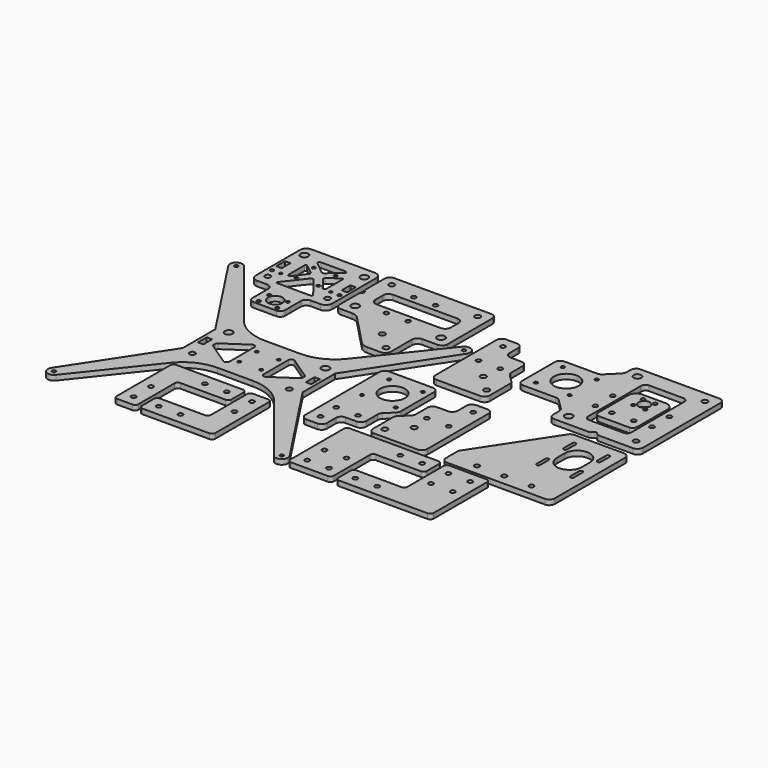
from build123d import *

# Parameters (mm, degrees)
F0_R     = 1.55
F0_R_2   = 6.75
F0_R_3   = 2.55
F0_R_4   = 1.6
F0_R_5   = 1.25
F0_R_6   = 1.5
F0_W     = 5
F0_H     = 10
F0_R_7   = 3.556
F1_DEPTH = 2.325
F0_R_8   = 2.15
F0_R_9   = 2.1
F0_R_10  = 11.5
F0_R_11  = 2.6
F0_R_12  = 1.65
F0_R_13  = 3.555
F0_R_14  = 2.125
F0_R_15  = 1.7531
F0_R_16  = 5.2592
F0_R_17  = 2.25


# Not quite as in the source:
# - ends of sketch curves that miss each other by under 0.0002 mm in the source are joined


with BuildPart() as f1:
    # F0 (on Top) → F1 (new body, symmetric)
    with BuildSketch(Plane.XY):
        with BuildLine():
            ThreePointArc((-173.037736, 133.310467), (-177.2803766871, 131.5531076871), (-179.037736, 127.310467))
            Line((-179.037736, 127.310467), (-179.037736, 76.929897))
            ThreePointArc((-179.037736, 76.929897), (-177.2803766871, 72.6872563129), (-173.037736, 70.929897))
            Line((-173.037736, 70.929897), (-164.037736, 70.929897))
            ThreePointArc((-164.037736, 70.929897), (-160.5022020941, 69.4654309059), (-159.037736, 65.929897))
            Line((-159.037736, 65.929897), (-159.037736, 47.929897))
            ThreePointArc((-159.037736, 47.929897), (-157.7197165153, 44.7479164847), (-154.537736, 43.429897))
            Line((-154.537736, 43.429897), (-133.537736, 43.429897))
            ThreePointArc((-133.537736, 43.429897), (-130.3557554847, 44.7479164847), (-129.037736, 47.929897))
            Line((-129.037736, 47.929897), (-129.037736, 65.929897))
            ThreePointArc((-129.037736, 65.929897), (-127.5732699059, 69.4654309059), (-124.037736, 70.929897))
            Line((-124.037736, 70.929897), (-115.037736, 70.929897))
            ThreePointArc((-115.037736, 70.929897), (-110.7950953129, 72.6872563129), (-109.037736, 76.929897))
            Line((-109.037736, 76.929897), (-109.037736, 127.310467))
            ThreePointArc((-109.037736, 127.310467), (-110.7950953129, 131.5531076871), (-115.037736, 133.310467))
            Line((-115.037736, 133.310467), (-173.037736, 133.310467))
        make_face()
        with Locations((-152.537736, 47.029897)):
            Circle(F0_R, mode=Mode.SUBTRACT)
        with Locations((-135.537736, 47.029897)):
            Circle(F0_R, mode=Mode.SUBTRACT)
        with Locations((-152.537736, 59.029897)):
            Circle(F0_R, mode=Mode.SUBTRACT)
        with Locations((-144.037736, 55.429897)):
            Circle(F0_R_2, mode=Mode.SUBTRACT)
        with Locations((-135.537736, 59.029897)):
            Circle(F0_R, mode=Mode.SUBTRACT)
        with Locations((-171.537736, 81.114382)):
            Circle(F0_R_3, mode=Mode.SUBTRACT)
        with Locations((-174.992762, 90.275039)):
            Circle(F0_R_4, mode=Mode.SUBTRACT)
        with Locations((-166.992762, 90.275039)):
            Circle(F0_R_5, mode=Mode.SUBTRACT)
        with Locations((-154.037736, 92.120182)):
            Circle(F0_R_6, mode=Mode.SUBTRACT)
        with BuildLine():
            Line((-161.537736, 92.349506), (-161.537736, 110.969423))
            ThreePointArc((-161.537736, 110.969423), (-160.9765059421, 111.8680224313), (-159.9227741241, 111.7579798408))
            Line((-159.9227741241, 111.7579798408), (-150.887467, 104.711742))
            ThreePointArc((-150.887467, 104.711742), (-150.3212527314, 103.7130323531), (-150.6270730647, 102.6064640505))
            Line((-150.6270730647, 102.6064640505), (-151.006303, 102.120182))
            Line((-151.006303, 102.120182), (-158.828462, 91.462006))
            ThreePointArc((-158.828462, 91.462006), (-160.5046883222, 90.9240392242), (-161.537736, 92.349506))
        make_face(mode=Mode.SUBTRACT)
        with Locations((-116.537736, 81.114382)):
            Circle(F0_R_3, mode=Mode.SUBTRACT)
        with BuildLine():
            Line((-128.58573, 76.929897), (-159.489741, 76.929897))
            ThreePointArc((-159.489741, 76.929897), (-160.3883402583, 77.4911267036), (-160.2782983258, 78.544858254))
            Line((-160.2782983258, 78.544858254), (-145.61485, 97.347622))
            ThreePointArc((-145.61485, 97.347622), (-144.0377356925, 98.1177), (-142.4606209703, 97.3476220232))
            Line((-142.4606209703, 97.3476220232), (-127.797173, 78.544858))
            ThreePointArc((-127.797173, 78.544858), (-127.6871307417, 77.4911267036), (-128.58573, 76.929897))
        make_face(mode=Mode.SUBTRACT)
        with Locations((-134.037736, 92.120182)):
            Circle(F0_R_6, mode=Mode.SUBTRACT)
        with BuildLine():
            Line((-129.220572, 91.210621), (-137.85836, 102.286753))
            ThreePointArc((-137.85836, 102.286753), (-138.1641792309, 103.3933216583), (-137.5979649495, 104.3920309353))
            Line((-137.5979649495, 104.3920309353), (-128.152697, 111.75798))
            ThreePointArc((-128.152697, 111.75798), (-127.0989657036, 111.8680222583), (-126.537736, 110.969423))
            Line((-126.537736, 110.969423), (-126.537736, 92.133063))
            ThreePointArc((-126.537736, 92.133063), (-127.5500136932, 90.7145683925), (-129.220572, 91.210621))
        make_face(mode=Mode.SUBTRACT)
        with Locations((-120.992762, 90.275039)):
            Circle(F0_R_5, mode=Mode.SUBTRACT)
        with Locations((-112.992762, 90.275039)):
            Circle(F0_R_4, mode=Mode.SUBTRACT)
        with Locations((-174.037736, 102.120182)):
            Rectangle(F0_W, F0_H, mode=Mode.SUBTRACT)
        with Locations((-154.037736, 112.120182)):
            Circle(F0_R_6, mode=Mode.SUBTRACT)
        with Locations((-171.537736, 123.125982)):
            Circle(F0_R_7, mode=Mode.SUBTRACT)
        with BuildLine():
            Line((-155.334091, 121.809978), (-132.741381, 121.809978))
            ThreePointArc((-132.741381, 121.809978), (-131.3304796262, 120.8192493553), (-131.7833387935, 119.1557877512))
            Line((-131.7833387935, 119.1557877512), (-142.760347, 110.044269))
            ThreePointArc((-142.760347, 110.044269), (-144.0377356153, 109.58319), (-145.3151243278, 110.044268605))
            Line((-145.3151243278, 110.044268605), (-156.292132, 119.155788))
            ThreePointArc((-156.292132, 119.155788), (-156.7449925044, 120.8192489935), (-155.334091, 121.809978))
        make_face(mode=Mode.SUBTRACT)
        with Locations((-134.037736, 112.120182)):
            Circle(F0_R_6, mode=Mode.SUBTRACT)
        with Locations((-114.037736, 102.120182)):
            Rectangle(F0_W, F0_H, mode=Mode.SUBTRACT)
        with Locations((-116.537736, 123.125982)):
            Circle(F0_R_7, mode=Mode.SUBTRACT)
    extrude(amount=F1_DEPTH, both=True)


with BuildPart() as f1b:
    # F0 (on Top) → F1, piece 2 (new body, symmetric)
    with BuildSketch(Plane.XY):
        with BuildLine():
            Line((-116.875232, -87.385385), (-75.37523, -87.385385))
            ThreePointArc((-75.37523, -87.385385), (-73.2539096564, -86.5067053436), (-72.37523, -84.385385))
            Line((-72.37523, -84.385385), (-72.37523, -70.385385))
            ThreePointArc((-72.37523, -70.385385), (-73.2539096564, -68.2640646564), (-75.37523, -67.385385))
            Line((-75.37523, -67.385385), (-136.87523, -67.385385))
            ThreePointArc((-136.87523, -67.385385), (-138.9965503436, -68.2640646564), (-139.87523, -70.385385))
            Line((-139.87523, -70.385385), (-139.87523, -131.885385))
            ThreePointArc((-139.87523, -131.885385), (-138.9965503436, -134.0067053436), (-136.87523, -134.885385))
            Line((-136.87523, -134.885385), (-122.875232, -134.885385))
            ThreePointArc((-122.875232, -134.885385), (-120.7539116564, -134.0067053436), (-119.875232, -131.885385))
            Line((-119.875232, -131.885385), (-119.875232, -90.385385))
            ThreePointArc((-119.875232, -90.385385), (-118.9965523436, -88.2640646564), (-116.875232, -87.385385))
        make_face()
        with Locations((-129.875231, -124.885385)):
            Circle(F0_R_8, mode=Mode.SUBTRACT)
        with Locations((-129.875231, -104.885385)):
            Circle(F0_R_8, mode=Mode.SUBTRACT)
        with Locations((-102.37523, -77.385385)):
            Circle(F0_R_8, mode=Mode.SUBTRACT)
        with Locations((-82.37523, -77.385385)):
            Circle(F0_R_8, mode=Mode.SUBTRACT)
    extrude(amount=F1_DEPTH, both=True)


with BuildPart() as f1c:
    # F0 (on Top) → F1, piece 3 (new body, symmetric)
    with BuildSketch(Plane.XY):
        with BuildLine():
            ThreePointArc((-51.875233, -135.385385), (-49.7539126564, -134.5067053436), (-48.875233, -132.385385))
            Line((-48.875233, -132.385385), (-48.875233, -70.885386))
            ThreePointArc((-48.875233, -70.885386), (-49.7539126564, -68.7640656564), (-51.875233, -67.885386))
            Line((-51.875233, -67.885386), (-65.875232, -67.885386))
            ThreePointArc((-65.875232, -67.885386), (-67.9965523436, -68.7640656564), (-68.875232, -70.885386))
            Line((-68.875232, -70.885386), (-68.875232, -112.385385))
            ThreePointArc((-68.875232, -112.385385), (-69.7539116564, -114.5067053436), (-71.875232, -115.385385))
            Line((-71.875232, -115.385385), (-113.375233, -115.385385))
            ThreePointArc((-113.375233, -115.385385), (-115.4965533436, -116.2640646564), (-116.375233, -118.385385))
            Line((-116.375233, -118.385385), (-116.375233, -132.385385))
            ThreePointArc((-116.375233, -132.385385), (-115.4965533436, -134.5067053436), (-113.375233, -135.385385))
            Line((-113.375233, -135.385385), (-51.875233, -135.385385))
        make_face()
        with Locations((-106.375233, -125.385385)):
            Circle(F0_R_8, mode=Mode.SUBTRACT)
        with Locations((-86.375233, -125.385385)):
            Circle(F0_R_8, mode=Mode.SUBTRACT)
        with Locations((-58.875232, -97.885386)):
            Circle(F0_R_8, mode=Mode.SUBTRACT)
        with Locations((-58.875232, -77.885386)):
            Circle(F0_R_8, mode=Mode.SUBTRACT)
    extrude(amount=F1_DEPTH, both=True)


with BuildPart() as f1d:
    # F0 (on Top) → F1, piece 4 (new body, symmetric)
    with BuildSketch(Plane.XY):
        with BuildLine():
            Line((33.884182, -23.014414), (33.884182, 14.914518))
            ThreePointArc((33.884182, 14.914518), (32.4197159059, 18.4500519059), (28.884182, 19.914518))
            Line((28.884182, 19.914518), (-11.115818, 19.914518))
            ThreePointArc((-11.115818, 19.914518), (-14.6513519059, 18.4500519059), (-16.115818, 14.914518))
            Line((-16.115818, 14.914518), (-16.115818, -70.085482))
            ThreePointArc((-16.115818, -70.085482), (-14.6513519059, -73.6210159059), (-11.115818, -75.085482))
            Line((-11.115818, -75.085482), (-1.115818, -75.085482))
            ThreePointArc((-1.115818, -75.085482), (2.4197159059, -73.6210159059), (3.884182, -70.085482))
            Line((3.884182, -70.085482), (3.884182, -60.085482))
            ThreePointArc((3.884182, -60.085482), (5.3486480941, -56.5499480941), (8.884182, -55.085482))
            Line((8.884182, -55.085482), (18.884182, -55.085482))
            ThreePointArc((18.884182, -55.085482), (22.4197159059, -53.6210159059), (23.884182, -50.085482))
            Line((23.884182, -50.085482), (23.884182, -37.15655))
            ThreePointArc((23.884182, -37.15655), (24.2647843374, -35.2431328382), (25.3486480941, -33.6210160941))
            Line((25.3486480941, -33.6210160941), (32.419716, -26.549948))
            ThreePointArc((32.419716, -26.549948), (33.5035796626, -24.9278311618), (33.884182, -23.014414))
        make_face()
        with Locations((-6.115818, -65.085482)):
            Circle(F0_R_9, mode=Mode.SUBTRACT)
        with Locations((-6.115818, -47.085482)):
            Circle(F0_R_9, mode=Mode.SUBTRACT)
        with Locations((-3.615818, -20.585482)):
            Circle(F0_R_4, mode=Mode.SUBTRACT)
        with Locations((13.884182, -47.085482)):
            Circle(F0_R_9, mode=Mode.SUBTRACT)
        with Locations((27.384182, -20.585482)):
            Circle(F0_R_4, mode=Mode.SUBTRACT)
        with Locations((11.884182, -5.085482)):
            Circle(F0_R_10, mode=Mode.SUBTRACT)
        with Locations((-3.615818, 10.414518)):
            Circle(F0_R_4, mode=Mode.SUBTRACT)
        with Locations((27.384182, 10.414518)):
            Circle(F0_R_4, mode=Mode.SUBTRACT)
    extrude(amount=F1_DEPTH, both=True)


with BuildPart() as f1e:
    # F0 (on Top) → F1, piece 5 (new body, symmetric)
    with BuildSketch(Plane.XY):
        with BuildLine():
            Line((45.248714, -6.784818), (45.248714, -19.713751))
            ThreePointArc((45.248714, -19.713751), (44.8681117979, -21.6271678352), (43.7842484059, -23.2492844059))
            Line((43.7842484059, -23.2492844059), (36.71318, -30.320352))
            ThreePointArc((36.71318, -30.320352), (35.6293163374, -31.9424688382), (35.248714, -33.855886))
            Line((35.248714, -33.855886), (35.248714, -56.784818))
            ThreePointArc((35.248714, -56.784818), (36.7131800941, -60.3203519059), (40.248714, -61.784818))
            Line((40.248714, -61.784818), (80.248714, -61.784818))
            ThreePointArc((80.248714, -61.784818), (83.7842479059, -60.3203519059), (85.248714, -56.784818))
            Line((85.248714, -56.784818), (85.248714, 13.215182))
            ThreePointArc((85.248714, 13.215182), (83.7842479059, 16.7507159059), (80.248714, 18.215182))
            Line((80.248714, 18.215182), (70.248714, 18.215182))
            ThreePointArc((70.248714, 18.215182), (66.7131800941, 16.7507159059), (65.248714, 13.215182))
            Line((65.248714, 13.215182), (65.248714, 3.215182))
            ThreePointArc((65.248714, 3.215182), (63.7842479059, -0.3203519059), (60.248714, -1.784818))
            Line((60.248714, -1.784818), (50.248714, -1.784818))
            ThreePointArc((50.248714, -1.784818), (46.7131800941, -3.2492840941), (45.248714, -6.784818))
        make_face()
        with Locations((42.248714, -51.784818)):
            Circle(F0_R_11, mode=Mode.SUBTRACT)
        with Locations((57.248714, -36.784818)):
            Circle(F0_R_11, mode=Mode.SUBTRACT)
        with Locations((55.248714, -19.784818)):
            Circle(F0_R_9, mode=Mode.SUBTRACT)
        with Locations((75.248714, -19.784818)):
            Circle(F0_R_9, mode=Mode.SUBTRACT)
        with Locations((75.248714, 8.215182)):
            Circle(F0_R_9, mode=Mode.SUBTRACT)
    extrude(amount=F1_DEPTH, both=True)


with BuildPart() as f1f:
    # F0 (on Top) → F1, piece 6 (new body, symmetric)
    with BuildSketch(Plane.XY):
        with BuildLine():
            Line((68.248714, 36.215182), (68.248714, 59.144114))
            ThreePointArc((68.248714, 59.144114), (67.8681116626, 61.0575311618), (66.7842479059, 62.6796479059))
            Line((66.7842479059, 62.6796479059), (59.71318, 69.750716))
            ThreePointArc((59.71318, 69.750716), (58.6293162021, 71.3728321648), (58.248714, 73.286249))
            Line((58.248714, 73.286249), (58.248714, 86.215182))
            ThreePointArc((58.248714, 86.215182), (56.7842479059, 89.7507159059), (53.248714, 91.215182))
            Line((53.248714, 91.215182), (43.248714, 91.215182))
            ThreePointArc((43.248714, 91.215182), (39.7131800941, 92.6796480941), (38.248714, 96.215182))
            Line((38.248714, 96.215182), (38.248714, 106.215182))
            ThreePointArc((38.248714, 106.215182), (36.7842479059, 109.7507159059), (33.248714, 111.215182))
            Line((33.248714, 111.215182), (23.248714, 111.215182))
            ThreePointArc((23.248714, 111.215182), (19.7131800941, 109.7507159059), (18.248714, 106.215182))
            Line((18.248714, 106.215182), (18.248714, 36.215182))
            ThreePointArc((18.248714, 36.215182), (19.7131800941, 32.6796480941), (23.248714, 31.215182))
            Line((23.248714, 31.215182), (63.248714, 31.215182))
            ThreePointArc((63.248714, 31.215182), (66.7842479059, 32.6796480941), (68.248714, 36.215182))
        make_face()
        with Locations((46.248714, 56.215182)):
            Circle(F0_R_11, mode=Mode.SUBTRACT)
        with Locations((61.248714, 41.215182)):
            Circle(F0_R_11, mode=Mode.SUBTRACT)
        with Locations((28.248714, 73.215182)):
            Circle(F0_R_9, mode=Mode.SUBTRACT)
        with Locations((48.248714, 73.215182)):
            Circle(F0_R_9, mode=Mode.SUBTRACT)
        with Locations((28.248714, 101.215182)):
            Circle(F0_R_9, mode=Mode.SUBTRACT)
    extrude(amount=F1_DEPTH, both=True)


with BuildPart() as f1g:
    # F0 (on Top) → F1, piece 7 (new body, symmetric)
    with BuildSketch(Plane.XY):
        with BuildLine():
            Line((61.845002, -86.57472), (103.338126, -86.669826))
            ThreePointArc((103.338126, -86.669826), (105.4638899166, -85.7935829846), (106.345002, -83.669833))
            Line((106.345002, -83.669833), (106.345002, -69.57472))
            ThreePointArc((106.345002, -69.57472), (105.4663223436, -67.4533996564), (103.345002, -66.57472))
            Line((103.345002, -66.57472), (21.845002, -66.57472))
            ThreePointArc((21.845002, -66.57472), (19.7236816564, -67.4533996564), (18.845002, -69.57472))
            Line((18.845002, -69.57472), (18.845002, -131.074719))
            ThreePointArc((18.845002, -131.074719), (19.7236816564, -133.1960393436), (21.845002, -134.074719))
            Line((21.845002, -134.074719), (55.845002, -134.074719))
            ThreePointArc((55.845002, -134.074719), (57.9663223436, -133.1960393436), (58.845002, -131.074719))
            Line((58.845002, -131.074719), (58.845002, -89.57472))
            ThreePointArc((58.845002, -89.57472), (59.7236816564, -87.4533996564), (61.845002, -86.57472))
        make_face()
        with Locations((28.845003, -124.074719)):
            Circle(F0_R_8, mode=Mode.SUBTRACT)
        with Locations((48.845003, -124.074719)):
            Circle(F0_R_8, mode=Mode.SUBTRACT)
        with Locations((28.845003, -104.074719)):
            Circle(F0_R_8, mode=Mode.SUBTRACT)
        with Locations((48.845003, -104.074719)):
            Circle(F0_R_8, mode=Mode.SUBTRACT)
        with Locations((76.345002, -76.622277)):
            Circle(F0_R_8, mode=Mode.SUBTRACT)
        with Locations((96.345002, -76.622277)):
            Circle(F0_R_8, mode=Mode.SUBTRACT)
    extrude(amount=F1_DEPTH, both=True)


with BuildPart() as f1h:
    # F0 (on Top) → F1, piece 8 (new body, symmetric)
    with BuildSketch(Plane.XY):
        with BuildLine():
            ThreePointArc((147.845003, -134.574719), (149.9663233436, -133.6960393436), (150.845003, -131.574719))
            Line((150.845003, -131.574719), (150.845003, -70.074719))
            ThreePointArc((150.845003, -70.074719), (149.9663233436, -67.9533986564), (147.845003, -67.074719))
            Line((147.845003, -67.074719), (113.845003, -67.074719))
            ThreePointArc((113.845003, -67.074719), (111.7236826564, -67.9533986564), (110.845003, -70.074719))
            Line((110.845003, -70.074719), (110.845003, -111.574719))
            ThreePointArc((110.845003, -111.574719), (109.9663233436, -113.6960393436), (107.845003, -114.574719))
            Line((107.845003, -114.574719), (66.351879, -114.479613))
            ThreePointArc((66.351879, -114.479613), (64.2261150842, -115.3558550146), (63.345003, -117.479605))
            Line((63.345003, -117.479605), (63.345003, -131.574719))
            ThreePointArc((63.345003, -131.574719), (64.2236826564, -133.6960393436), (66.345003, -134.574719))
            Line((66.345003, -134.574719), (147.845003, -134.574719))
        make_face()
        with Locations((73.345003, -124.527162)):
            Circle(F0_R_8, mode=Mode.SUBTRACT)
        with Locations((93.345003, -124.527162)):
            Circle(F0_R_8, mode=Mode.SUBTRACT)
        with Locations((120.845002, -97.074719)):
            Circle(F0_R_8, mode=Mode.SUBTRACT)
        with Locations((140.845003, -97.074719)):
            Circle(F0_R_8, mode=Mode.SUBTRACT)
        with Locations((120.845002, -77.074719)):
            Circle(F0_R_8, mode=Mode.SUBTRACT)
        with Locations((140.845003, -77.074719)):
            Circle(F0_R_8, mode=Mode.SUBTRACT)
    extrude(amount=F1_DEPTH, both=True)


with BuildPart() as f1i:
    # F0 (on Top) → F1, piece 9 (new body, symmetric)
    with BuildSketch(Plane.XY):
        with BuildLine():
            Line((-142.147129, 16.845171), (-194.538469, 82.780025))
            ThreePointArc((-194.538469, 82.780025), (-202.3509475419, 83.8542157394), (-203.7782368598, 76.098472092))
            Line((-203.7782368598, 76.098472092), (-149.506709, -6.606183))
            Line((-149.506709, -6.606183), (-149.506709, -43.934666))
            Line((-149.506709, -43.934666), (-203.778237, -126.639321))
            ThreePointArc((-203.778237, -126.639321), (-202.3508964553, -134.3951006812), (-194.538390534, -133.3207753703))
            Line((-194.538390534, -133.3207753703), (-142.150034, -67.386707))
            ThreePointArc((-142.150034, -67.386707), (-128.2198123066, -56.2471766972), (-110.832298, -52.270424))
            Line((-110.832298, -52.270424), (-78.181167, -52.270424))
            ThreePointArc((-78.181167, -52.270424), (-60.7936526934, -56.2471766972), (-46.8634306076, -67.3867066882))
            Line((-46.8634306076, -67.3867066882), (5.524926, -133.320775))
            ThreePointArc((5.524926, -133.320775), (13.3374324255, -134.3951007027), (14.7647730175, -126.6393203323))
            Line((14.7647730175, -126.6393203323), (-39.506756, -43.934666))
            Line((-39.506756, -43.934666), (-39.506756, -6.606183))
            Line((-39.506756, -6.606183), (14.764772, 76.098472))
            ThreePointArc((14.764772, 76.098472), (13.3374835121, 83.8542157609), (5.5250040662, 82.7800249474))
            Line((5.5250040662, 82.7800249474), (-46.866336, 16.845171))
            ThreePointArc((-46.866336, 16.845171), (-60.7964071972, 5.7061378002), (-78.183526, 1.729576))
            Line((-78.183526, 1.729576), (-110.829938, 1.729576))
            ThreePointArc((-110.829938, 1.729576), (-128.217057083, 5.7061379354), (-142.147129, 16.845171))
        make_face()
        with Locations((-199.006732, -129.770424)):
            Circle(F0_R_12, mode=Mode.SUBTRACT)
        with Locations((-138.951709, -46.078176)):
            Circle(F0_R_3, mode=Mode.SUBTRACT)
        with Locations((-104.506732, -35.270424)):
            Circle(F0_R_6, mode=Mode.SUBTRACT)
        with Locations((-144.006709, -25.270424)):
            Rectangle(F0_W, F0_H, mode=Mode.SUBTRACT)
        with BuildLine():
            Line((-114.088685, -41.643578), (-134.310491, -28.013687))
            ThreePointArc((-134.310491, -28.013687), (-135.1203767533, -27.1146727652), (-135.413205, -25.940623))
            Line((-135.413205, -25.940623), (-135.413205, -24.600248))
            ThreePointArc((-135.413205, -24.600248), (-135.1203770793, -23.4261988475), (-134.3104918701, -22.5271851928))
            Line((-134.3104918701, -22.5271851928), (-114.088687, -8.897275))
            ThreePointArc((-114.088687, -8.897275), (-111.5173508475, -8.7631659207), (-110.1914, -10.970338))
            Line((-110.1914, -10.970338), (-110.1914, -39.570514))
            ThreePointArc((-110.1914, -39.570514), (-111.5173498687, -41.7776855586), (-114.088685, -41.643578))
        make_face(mode=Mode.SUBTRACT)
        with Locations((-138.951709, -4.459606)):
            Circle(F0_R_13, mode=Mode.SUBTRACT)
        with Locations((-104.506732, -15.270424)):
            Circle(F0_R_6, mode=Mode.SUBTRACT)
        with Locations((-84.506732, -35.270424)):
            Circle(F0_R_6, mode=Mode.SUBTRACT)
        with Locations((-50.061756, -46.078176)):
            Circle(F0_R_3, mode=Mode.SUBTRACT)
        with BuildLine():
            Line((-74.924778, -8.897275), (-54.702973, -22.527185))
            ThreePointArc((-54.702973, -22.527185), (-53.8930879207, -23.4261988475), (-53.60026, -24.600248))
            Line((-53.60026, -24.600248), (-53.60026, -25.940623))
            ThreePointArc((-53.60026, -25.940623), (-53.8930882467, -27.1146727652), (-54.702974281, -28.0136865831))
            Line((-54.702974281, -28.0136865831), (-74.92478, -41.643578))
            ThreePointArc((-74.92478, -41.643578), (-77.4961151313, -41.7776855586), (-78.822065, -39.570514))
            Line((-78.822065, -39.570514), (-78.822065, -10.970338))
            ThreePointArc((-78.822065, -10.970338), (-77.4961141525, -8.7631659207), (-74.924778, -8.897275))
        make_face(mode=Mode.SUBTRACT)
        with Locations((-84.506732, -15.270424)):
            Circle(F0_R_6, mode=Mode.SUBTRACT)
        with Locations((-45.006756, -25.270424)):
            Rectangle(F0_W, F0_H, mode=Mode.SUBTRACT)
        with Locations((-50.061756, -4.459606)):
            Circle(F0_R_13, mode=Mode.SUBTRACT)
        with Locations((9.993268, -129.770424)):
            Circle(F0_R_12, mode=Mode.SUBTRACT)
        with Locations((-199.006732, 79.229576)):
            Circle(F0_R_12, mode=Mode.SUBTRACT)
        with Locations((9.993268, 79.229576)):
            Circle(F0_R_12, mode=Mode.SUBTRACT)
    extrude(amount=F1_DEPTH, both=True)


with BuildPart() as f1j:
    # F0 (on Top) → F1, piece 10 (new body, symmetric)
    with BuildSketch(Plane.XY):
        with BuildLine():
            ThreePointArc((-103.847813, 108.4256), (-103.6955722003, 107.6602334619), (-103.2620270624, 107.0113869376))
            Line((-103.2620270624, 107.0113869376), (-102.452101, 106.201461))
            ThreePointArc((-102.452101, 106.201461), (-101.866314, 104.787247), (-102.4521009376, 103.3730329376))
            Line((-102.4521009376, 103.3730329376), (-103.262027, 102.563107))
            ThreePointArc((-103.262027, 102.563107), (-103.6955722003, 101.9142605381), (-103.847813, 101.148894))
            Line((-103.847813, 101.148894), (-103.847813, 79.096962))
            ThreePointArc((-103.847813, 79.096962), (-102.3833469059, 75.5614280941), (-98.847813, 74.096962))
            Line((-98.847813, 74.096962), (-88.746397, 74.096962))
            ThreePointArc((-88.746397, 74.096962), (-84.8220228823, 73.2947491134), (-81.5272854623, 71.0168195568))
            Line((-81.5272854623, 71.0168195568), (-54.432208, 42.749997))
            ThreePointArc((-54.432208, 42.749997), (-51.1374704497, 40.4720670282), (-47.213096, 39.669854))
            Line((-47.213096, 39.669854), (-34.479747, 39.669854))
            ThreePointArc((-34.479747, 39.669854), (-30.9442130941, 41.1343200941), (-29.479747, 44.669854))
            Line((-29.479747, 44.669854), (-29.479747, 69.096962))
            ThreePointArc((-29.479747, 69.096962), (-28.0152809059, 72.6324959059), (-24.479747, 74.096962))
            Line((-24.479747, 74.096962), (-9.957813, 74.096962))
            ThreePointArc((-9.957813, 74.096962), (-6.4222790941, 75.5614280941), (-4.957813, 79.096962))
            Line((-4.957813, 79.096962), (-4.957813, 130.477532))
            ThreePointArc((-4.957813, 130.477532), (-6.4222790941, 134.0130659059), (-9.957813, 135.477532))
            Line((-9.957813, 135.477532), (-98.847813, 135.477532))
            ThreePointArc((-98.847813, 135.477532), (-102.3833469059, 134.0130659059), (-103.847813, 130.477532))
            Line((-103.847813, 130.477532), (-103.847813, 108.4256))
        make_face()
        with Locations((-51.479747, 62.527664)):
            Circle(F0_R_11, mode=Mode.SUBTRACT)
        with Locations((-35.979747, 47.527664)):
            Circle(F0_R_11, mode=Mode.SUBTRACT)
        with Locations((-93.847813, 84.287247)):
            Circle(F0_R_13, mode=Mode.SUBTRACT)
        with Locations((-69.482813, 89.56358)):
            Circle(F0_R_9, mode=Mode.SUBTRACT)
        with Locations((-14.957813, 84.287247)):
            Circle(F0_R_13, mode=Mode.SUBTRACT)
        with Locations((-49.482813, 89.56358)):
            Circle(F0_R_9, mode=Mode.SUBTRACT)
        with BuildLine():
            Line((-83.452813, 114.812247), (-24.397813, 114.812247))
            ThreePointArc((-24.397813, 114.812247), (-20.8057105516, 113.3243494484), (-19.317813, 109.732247))
            Line((-19.317813, 109.732247), (-19.317813, 100.842247))
            ThreePointArc((-19.317813, 100.842247), (-20.8057105516, 97.2501445516), (-24.397813, 95.762247))
            Line((-24.397813, 95.762247), (-83.452813, 95.762247))
            ThreePointArc((-83.452813, 95.762247), (-87.0449154484, 97.2501445516), (-88.532813, 100.842247))
            Line((-88.532813, 100.842247), (-88.532813, 109.732247))
            ThreePointArc((-88.532813, 109.732247), (-87.0449154484, 113.3243494484), (-83.452813, 114.812247))
        make_face(mode=Mode.SUBTRACT)
        with Locations((-93.847813, 126.287247)):
            Circle(F0_R_3, mode=Mode.SUBTRACT)
        with Locations((-69.482813, 121.06358)):
            Circle(F0_R_9, mode=Mode.SUBTRACT)
        with Locations((-49.482813, 121.06358)):
            Circle(F0_R_9, mode=Mode.SUBTRACT)
        with Locations((-14.957813, 126.287247)):
            Circle(F0_R_3, mode=Mode.SUBTRACT)
    extrude(amount=F1_DEPTH, both=True)


with BuildPart() as f1k:
    # F0 (on Top) → F1, piece 11 (new body, symmetric)
    with BuildSketch(Plane.XY):
        with BuildLine():
            ThreePointArc((166.4181374376, 36.8568824376), (167.0669841353, 36.423336935), (167.832351, 36.271096))
            Line((167.832351, 36.271096), (199.71384, 36.271096))
            ThreePointArc((199.71384, 36.271096), (203.2493739059, 37.7355620941), (204.71384, 41.271096))
            Line((204.71384, 41.271096), (204.71384, 130.161096))
            ThreePointArc((204.71384, 130.161096), (203.2493739059, 133.6966299059), (199.71384, 135.161096))
            Line((199.71384, 135.161096), (127.336337, 135.161096))
            ThreePointArc((127.336337, 135.161096), (123.8008030941, 133.6966299059), (122.336337, 130.161096))
            Line((122.336337, 130.161096), (122.336337, 125.969418))
            ThreePointArc((122.336337, 125.969418), (121.8529720314, 123.5393782045), (120.4764650605, 121.4792899395))
            Line((120.4764650605, 121.4792899395), (111.496209, 112.499034))
            ThreePointArc((111.496209, 112.499034), (109.4361207955, 111.1225269686), (107.006081, 110.639162))
            Line((107.006081, 110.639162), (77.267039, 110.639162))
            ThreePointArc((77.267039, 110.639162), (73.7315050941, 109.1746959059), (72.267039, 105.639162))
            Line((72.267039, 105.639162), (72.267039, 68.179162))
            ThreePointArc((72.267039, 68.179162), (73.7315050941, 64.6436280941), (77.267039, 63.179162))
            Line((77.267039, 63.179162), (107.006081, 63.179162))
            ThreePointArc((107.006081, 63.179162), (109.4361207955, 62.6957970314), (111.4962090605, 61.3192900605))
            Line((111.4962090605, 61.3192900605), (120.476465, 52.339034))
            ThreePointArc((120.476465, 52.339034), (121.8529720314, 50.2789457955), (122.336337, 47.848906))
            Line((122.336337, 47.848906), (122.336337, 41.271096))
            ThreePointArc((122.336337, 41.271096), (123.8008030941, 37.7355620941), (127.336337, 36.271096))
            Line((127.336337, 36.271096), (159.217826, 36.271096))
            ThreePointArc((159.217826, 36.271096), (159.9831925381, 36.4233367997), (160.6320390624, 36.8568819376))
            Line((160.6320390624, 36.8568819376), (162.110875, 38.335718))
            ThreePointArc((162.110875, 38.335718), (163.5250883536, 38.921504), (164.9393015624, 38.3357175624))
            Line((164.9393015624, 38.3357175624), (166.4181374376, 36.8568824376))
        make_face()
        with Locations((132.590337, 46.271096)):
            Circle(F0_R_13, mode=Mode.SUBTRACT)
        with Locations((194.45984, 46.271096)):
            Circle(F0_R_3, mode=Mode.SUBTRACT)
        with Locations((81.767039, 72.139162)):
            Circle(F0_R_4, mode=Mode.SUBTRACT)
        with Locations((97.267039, 87.639162)):
            Circle(F0_R_10, mode=Mode.SUBTRACT)
        with Locations((81.767039, 103.139162)):
            Circle(F0_R_4, mode=Mode.SUBTRACT)
        with Locations((112.767039, 72.139162)):
            Circle(F0_R_4, mode=Mode.SUBTRACT)
        with Locations((137.525088, 70.636096)):
            Circle(F0_R_9, mode=Mode.SUBTRACT)
        with Locations((137.525088, 90.636096)):
            Circle(F0_R_9, mode=Mode.SUBTRACT)
        with Locations((189.525088, 70.636096)):
            Circle(F0_R_9, mode=Mode.SUBTRACT)
        with BuildLine():
            Line((183.379638, 115.517939), (183.379638, 54.644253))
            ThreePointArc((183.379638, 54.644253), (182.2080651247, 51.8158258753), (179.379638, 50.644253))
            Line((179.379638, 50.644253), (147.670538, 50.644253))
            ThreePointArc((147.670538, 50.644253), (144.8421108753, 51.8158258753), (143.670538, 54.644253))
            Line((143.670538, 54.644253), (143.670538, 115.517939))
            ThreePointArc((143.670538, 115.517939), (144.8421108753, 118.3463661247), (147.670538, 119.517939))
            Line((147.670538, 119.517939), (179.379638, 119.517939))
            ThreePointArc((179.379638, 119.517939), (182.2080651247, 118.3463661247), (183.379638, 115.517939))
        make_face(mode=Mode.SUBTRACT)
        with Locations((189.525088, 90.636096)):
            Circle(F0_R_9, mode=Mode.SUBTRACT)
        with Locations((112.767039, 103.139162)):
            Circle(F0_R_4, mode=Mode.SUBTRACT)
        with Locations((132.590337, 125.161096)):
            Circle(F0_R_13, mode=Mode.SUBTRACT)
        with Locations((194.45984, 125.161096)):
            Circle(F0_R_3, mode=Mode.SUBTRACT)
    extrude(amount=F1_DEPTH, both=True)


with BuildPart() as f1l:
    # F0 (on Top) → F1, piece 12 (new body, symmetric)
    with BuildSketch(Plane.XY):
        with BuildLine():
            Line((145.670538, 98.425746), (145.670538, 63.746346))
            ThreePointArc((145.670538, 63.746346), (146.8421108753, 60.9179188753), (149.670538, 59.746346))
            Line((149.670538, 59.746346), (177.379638, 59.746346))
            ThreePointArc((177.379638, 59.746346), (180.2080651247, 60.9179188753), (181.379638, 63.746346))
            Line((181.379638, 63.746346), (181.379638, 98.425746))
            ThreePointArc((181.379638, 98.425746), (179.3293854683, 103.3754934683), (174.379638, 105.425746))
            Line((174.379638, 105.425746), (152.670538, 105.425746))
            ThreePointArc((152.670538, 105.425746), (147.7207905317, 103.3754934683), (145.670538, 98.425746))
        make_face()
        with Locations((153.362238, 69.793446)):
            Circle(F0_R_14, mode=Mode.SUBTRACT)
        with Locations((173.443138, 69.793446)):
            Circle(F0_R_14, mode=Mode.SUBTRACT)
        with Locations((157.824638, 88.705646)):
            Circle(F0_R_15, mode=Mode.SUBTRACT)
        with Locations((168.980638, 88.705646)):
            Circle(F0_R_15, mode=Mode.SUBTRACT)
        with Locations((163.455738, 94.389946)):
            Circle(F0_R_16, mode=Mode.SUBTRACT)
        with Locations((157.824638, 99.967946)):
            Circle(F0_R_15, mode=Mode.SUBTRACT)
        with Locations((168.980638, 99.967946)):
            Circle(F0_R_15, mode=Mode.SUBTRACT)
    extrude(amount=F1_DEPTH, both=True)


with BuildPart() as f1m:
    # F0 (on Top) → F1, piece 13 (new body, symmetric)
    with BuildSketch(Plane.XY):
        with BuildLine():
            ThreePointArc((199.455703, -64.5232), (202.9912369059, -63.0587339059), (204.455703, -59.5232))
            Line((204.455703, -59.5232), (204.455703, 21.0768))
            ThreePointArc((204.455703, 21.0768), (202.9912369059, 24.6123339059), (199.455703, 26.0768))
            Line((199.455703, 26.0768), (153.950513, 26.0768))
            ThreePointArc((153.950513, 26.0768), (151.578306248, 25.4782355755), (149.7740669236, 23.8258540503))
            Line((149.7740669236, 23.8258540503), (105.279256, -43.772032))
            ThreePointArc((105.279256, -43.772032), (104.6660143781, -45.0862042017), (104.455703, -46.521085))
            Line((104.455703, -46.521085), (104.455703, -59.5232))
            ThreePointArc((104.455703, -59.5232), (105.9201690941, -63.0587339059), (109.455703, -64.5232))
            Line((109.455703, -64.5232), (199.455703, -64.5232))
        make_face()
        with Locations((129.455703, -55.0232)):
            Circle(F0_R_17, mode=Mode.SUBTRACT)
        with Locations((154.455703, -55.0232)):
            Circle(F0_R_17, mode=Mode.SUBTRACT)
        with Locations((179.455703, -55.0232)):
            Circle(F0_R_17, mode=Mode.SUBTRACT)
        with BuildLine():
            Line((163.980445, -15.750068), (163.980445, -25.750068))
            ThreePointArc((163.980445, -25.750068), (162.355445, -27.375068), (160.730445, -25.750068))
            Line((160.730445, -25.750068), (160.730445, -15.750068))
            ThreePointArc((160.730445, -15.750068), (162.355445, -14.125068), (163.980445, -15.750068))
        make_face(mode=Mode.SUBTRACT)
        with BuildLine():
            Line((194.980445, -15.750068), (194.980445, -25.750068))
            ThreePointArc((194.980445, -25.750068), (193.355445, -27.375068), (191.730445, -25.750068))
            Line((191.730445, -25.750068), (191.730445, -15.750068))
            ThreePointArc((191.730445, -15.750068), (193.355445, -14.125068), (194.980445, -15.750068))
        make_face(mode=Mode.SUBTRACT)
        with BuildLine():
            Line((166.355703, -9.5232), (166.355703, -0.5232))
            ThreePointArc((166.355703, -0.5232), (177.855703, 10.9768), (189.355703, -0.5232))
            Line((189.355703, -0.5232), (189.355703, -9.5232))
            ThreePointArc((189.355703, -9.5232), (177.855703, -21.0232), (166.355703, -9.5232))
        make_face(mode=Mode.SUBTRACT)
        with BuildLine():
            Line((163.980445, 15.249932), (163.980445, 5.249932))
            ThreePointArc((163.980445, 5.249932), (162.355445, 3.624932), (160.730445, 5.249932))
            Line((160.730445, 5.249932), (160.730445, 15.249932))
            ThreePointArc((160.730445, 15.249932), (162.355445, 16.874932), (163.980445, 15.249932))
        make_face(mode=Mode.SUBTRACT)
        with BuildLine():
            Line((194.980445, 15.249932), (194.980445, 5.249932))
            ThreePointArc((194.980445, 5.249932), (193.355445, 3.624932), (191.730445, 5.249932))
            Line((191.730445, 5.249932), (191.730445, 15.249932))
            ThreePointArc((191.730445, 15.249932), (193.355445, 16.874932), (194.980445, 15.249932))
        make_face(mode=Mode.SUBTRACT)
    extrude(amount=F1_DEPTH, both=True)


solid = Compound([f1.part, f1b.part, f1c.part, f1d.part, f1e.part, f1f.part, f1g.part, f1h.part, f1i.part, f1j.part, f1k.part, f1l.part, f1m.part])
